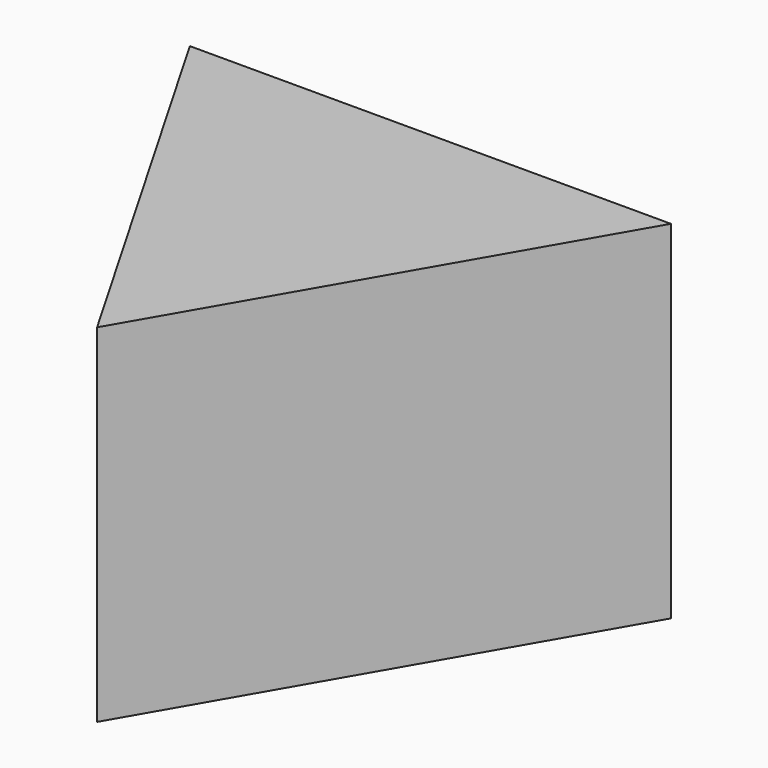
from build123d import *

# Parameters (mm, degrees)
F3_DEPTH = 25.4
F4_DEPTH = 43.688


# Not quite as in the source:
# - the program builds the solid bodies; features that only make, move or delete a surface that nothing else refers to are left out


with BuildPart() as f3:
    # F2 (on Top) → F3 (new body)
    with BuildSketch(Plane.XY):
        Polygon((27.2383972908, 95.090970397), (-68.4402532782, 95.090970397), (-20.6009279937, 12.2308284044), align=None)
    extrude(amount=F3_DEPTH)

    # F4 (add): a face of the model
    f4_faces = [f3.faces().sort_by_distance(p)[0] for p in [
        (-20.6009279937, 67.4709230661, 25.4),
    ]]
    extrude(f4_faces, amount=F4_DEPTH)


solid = f3.part
